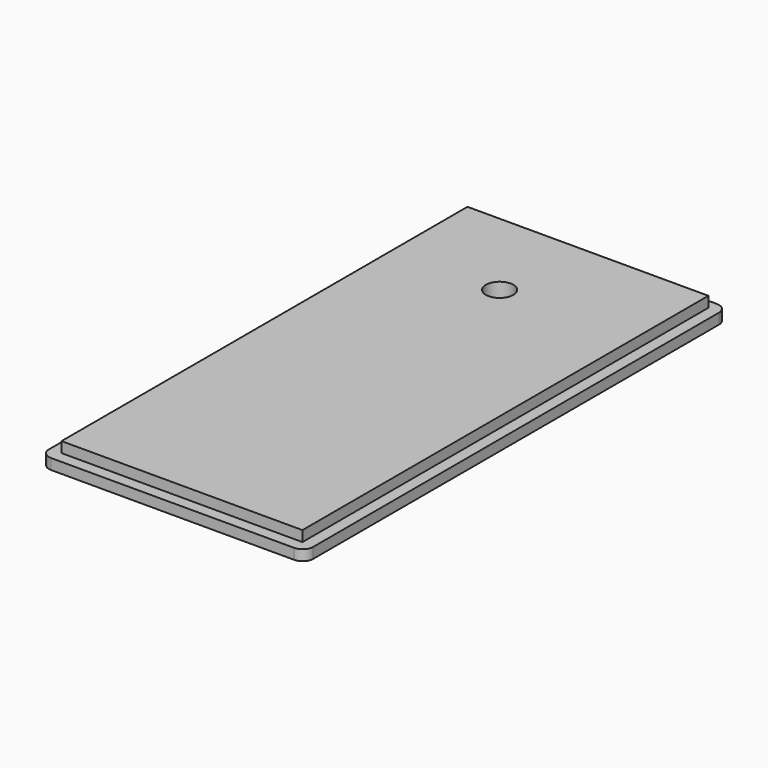
from build123d import *

# Parameters (mm, degrees)
F0_W         = 50
F0_H         = 100
F0_W_2       = 45.6
F0_H_2       = 96.0461332813
F0_R         = 2.6
F1_DEPTH     = 2
F2_DEPTH     = 4
F3_TEXT_SIZE = 9.2842241315
F4_DEPTH     = 5.5372
F5_R         = 2


# Not quite as in the source:
# - Text() gives the source's letters only with a copy of the font that has no kerning and outlines rounded to 1/6400 em; it was checked with that copy


with BuildPart() as f1:
    # F0 (on Top) → F1 (new body)
    with BuildSketch(Plane.XY):
        with Locations((87.2008845186, 10.6207997068)):
            Rectangle(F0_W, F0_H)
        with Locations((87.2008845186, 10.8438663475)):
            Rectangle(F0_W_2, F0_H_2, mode=Mode.SUBTRACT)
        with Locations((87.2008845186, 10.8438663475)):
            Rectangle(F0_W_2, F0_H_2)
        with Locations((84.7233086348, 41.0800652123)):
            Circle(F0_R, mode=Mode.SUBTRACT)
    extrude(amount=F1_DEPTH)

    # F0 (on Top) → F2 (join)
    with BuildSketch(Plane.XY):
        with Locations((87.2008845186, 10.8438663475)):
            Rectangle(F0_W_2, F0_H_2)
        with Locations((84.7233086348, 41.0800652123)):
            Circle(F0_R, mode=Mode.SUBTRACT)
    extrude(amount=F2_DEPTH)

    # F3 (on face) → F4 (join)
    with BuildSketch(Plane.XY.offset(4)):
        with Locations(Location((84.537781775, 34.3955355393), (0, 0, -90))):
            Text('MAGO GROUP', F3_TEXT_SIZE, font='Open Sans', text_align=(TextAlign.LEFT, TextAlign.BOTTOM))
    extrude(amount=-F4_DEPTH)

    # F5
    f5_edges = [f1.edges().sort_by_distance(p)[0] for p in [
        (112.200885, -39.3792, 1),
        (62.200885, -39.3792, 1),
        (62.200885, 60.6208, 1),
        (112.200885, 60.6208, 1),
    ]]
    fillet(f5_edges, radius=F5_R)


solid = f1.part
